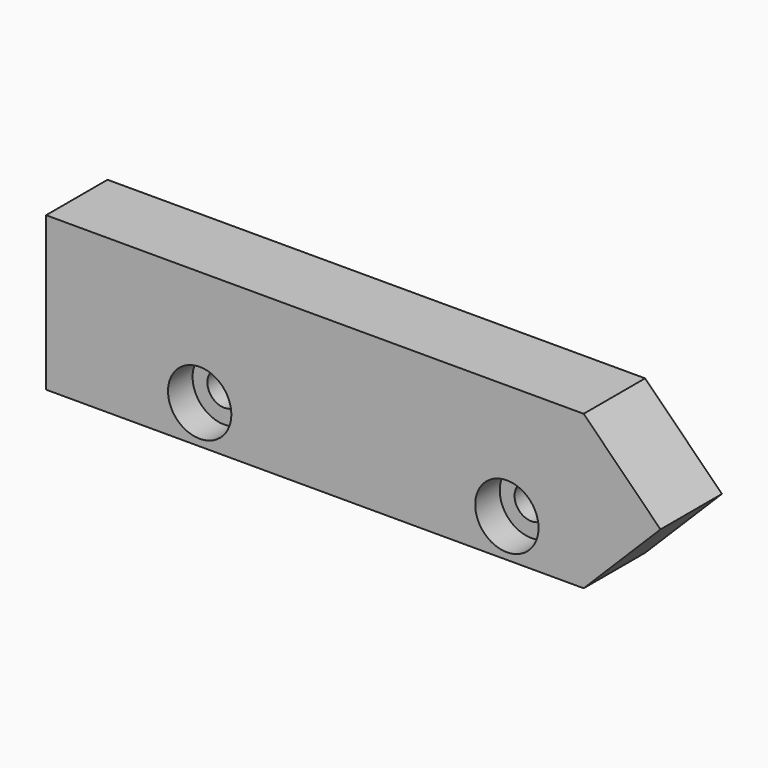
from build123d import *

# Parameters (mm, degrees)
F1_DEPTH       = 10
F3_D           = 4.4
F3_CBORE_D     = 8.25
F3_CBORE_DEPTH = 4


# Not quite as in the source:
# - a feature names something its author has since deleted; it is built from what else it names


with BuildPart() as f1:
    # F0 (on Front) → F1 (new body)
    with BuildSketch(Plane.XZ):
        Polygon((0, 10), (0, 0), (70, 0), (80, 10), align=None)
        Polygon((0, 20), (0, 10), (80, 10), (70, 20), align=None)
    extrude(amount=F1_DEPTH)

    # F3 (through all)
    with Locations(Plane.XZ.offset(10)):
        with Locations((20, 5), (60, 5)):
            CounterBoreHole(F3_D / 2, F3_CBORE_D / 2, F3_CBORE_DEPTH)


solid = f1.part
